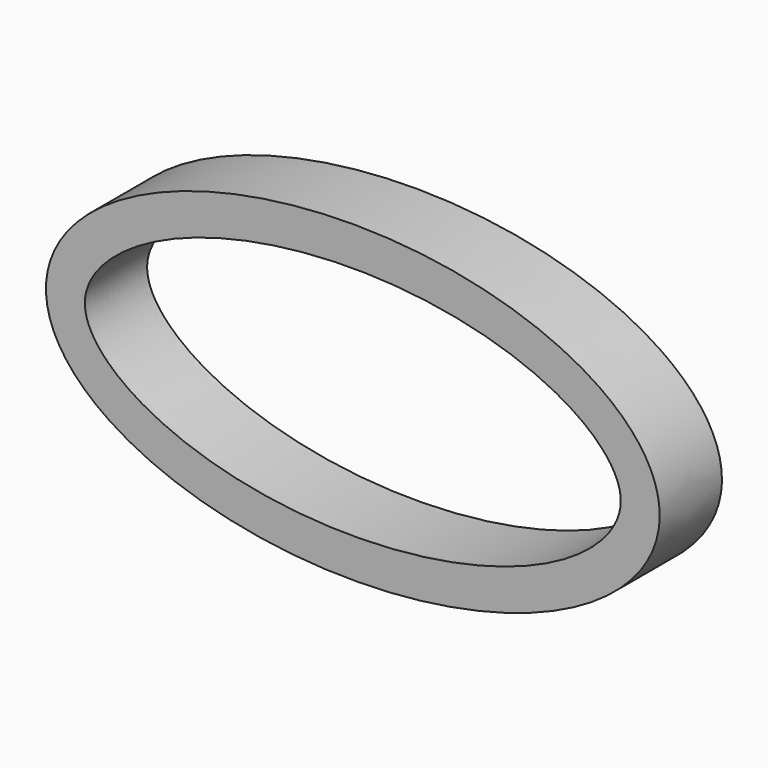
from build123d import *

# Parameters (mm, degrees)
F1_DEPTH = 12.7


# Not quite as in the source:
# - the dataset's text gives a spline's control points without its knots; the knots are read off the source's solid


with BuildPart() as f1:
    # F0 (on Front) → F1 (new body)
    with BuildSketch(Plane.XZ):
        with BuildLine():
            add(Edge.make_bspline(
                [(-50.0709774524, 20.9593381733), (-50.0709774524, -4.6166274828), (0, -4.6166274828), (50.0709774524, -4.6166274828), (50.0709774524, 20.9593381733)],
                knots=[3.1415926536, 3.1415926536, 3.1415926536, 4.7123889804, 4.7123889804, 6.2831853072, 6.2831853072, 6.2831853072], degree=2, weights=[1, 0.7071067812, 1, 0.7071067812, 1]))
            add(Edge.make_bspline(
                [(50.0709774524, 20.9593381733), (50.0709774524, 46.5353038293), (0, 46.5353038293), (-50.0709774524, 46.5353038293), (-50.0709774524, 20.9593381733)],
                knots=[0, 0, 0, 1.5707963268, 1.5707963268, 3.1415926536, 3.1415926536, 3.1415926536], degree=2, weights=[1, 0.7071067812, 1, 0.7071067812, 1]))
        make_face()
        with BuildLine():
            add(Edge.make_bspline(
                [(43.7209792435, 20.9593381733), (43.7209792435, 21.3941472691), (43.6378753479, 22.2637654609), (43.2418012763, 23.6381973689), (42.5148002756, 25.1317105062), (41.3984450909, 26.7351645875), (39.8553329616, 28.4111151874), (37.8704569502, 30.1115948), (35.8483113142, 31.5105625364), (34.0156886195, 32.5978275083), (32.5329973261, 33.3940879703), (30.9542874849, 34.1615740967), (28.741284138, 35.135430875), (25.7779291071, 36.2562859365), (21.9471588703, 37.4272897947), (17.8798753761, 38.4094991021), (13.6145661437, 39.1902890225), (9.1893604501, 39.7590330821), (5.3990551476, 40.0486007433), (2.3252694229, 40.1656128335), (0, 40.1951520139), (-2.3252694229, 40.1656128335), (-5.3990551476, 40.0486007433), (-9.1893604501, 39.7590330821), (-13.6145661437, 39.1902890225), (-17.8798753761, 38.4094991021), (-21.9471588703, 37.4272897947), (-25.7779291071, 36.2562859365), (-28.741284138, 35.135430875), (-30.9542874849, 34.1615740967), (-32.5329973261, 33.3940879703), (-34.0156886195, 32.5978275083), (-35.8483113142, 31.5105625364), (-37.8704569502, 30.1115948), (-39.8553329616, 28.4111151874), (-41.3984450909, 26.7351645875), (-42.5148002756, 25.1317105062), (-43.2418012763, 23.6381973689), (-43.6378753479, 22.2637654609), (-43.7625311913, 20.9593381733), (-43.6378753479, 19.6549108857), (-43.2418012763, 18.2804789776), (-42.5148002756, 16.7869658404), (-41.3984450909, 15.183511759), (-39.8553329616, 13.5075611592), (-37.8704569502, 11.8070815465), (-35.8483113142, 10.4081138101), (-34.0156886195, 9.3208488383), (-32.5329973261, 8.5245883762), (-30.9542874849, 7.7571022498), (-28.741284138, 6.7832454715), (-25.7779291071, 5.66239041), (-21.9471588703, 4.4913865518), (-17.8798753761, 3.5091772444), (-13.6145661437, 2.7283873241), (-9.1893604501, 2.1596432645), (-5.3990551476, 1.8700756033), (-2.3252694229, 1.753063513), (0, 1.7235243327), (2.3252694229, 1.753063513), (5.3990551476, 1.8700756033), (9.1893604501, 2.1596432645), (13.6145661437, 2.7283873241), (17.8798753761, 3.5091772444), (21.9471588703, 4.4913865518), (25.7779291071, 5.66239041), (28.741284138, 6.7832454715), (30.9542874849, 7.7571022498), (32.5329973261, 8.5245883762), (34.0156886195, 9.3208488383), (35.8483113142, 10.4081138101), (37.8704569502, 11.8070815465), (39.8553329616, 13.5075611592), (41.3984450909, 15.183511759), (42.5148002756, 16.7869658404), (43.2418012763, 18.2804789776), (43.6378753479, 19.6549108857), (43.7209792435, 20.5245290774), (43.7209792435, 20.9593381733)],
                knots=[0, 0, 0, 0, 0.015625, 0.03125, 0.046875, 0.0625, 0.078125, 0.09375, 0.109375, 0.1171875, 0.125, 0.1328125, 0.140625, 0.15625, 0.171875, 0.1875, 0.203125, 0.21875, 0.234375, 0.2421875, 0.25, 0.2578125, 0.265625, 0.28125, 0.296875, 0.3125, 0.328125, 0.34375, 0.359375, 0.3671875, 0.375, 0.3828125, 0.390625, 0.40625, 0.421875, 0.4375, 0.453125, 0.46875, 0.484375, 0.5, 0.515625, 0.53125, 0.546875, 0.5625, 0.578125, 0.59375, 0.609375, 0.6171875, 0.625, 0.6328125, 0.640625, 0.65625, 0.671875, 0.6875, 0.703125, 0.71875, 0.734375, 0.7421875, 0.75, 0.7578125, 0.765625, 0.78125, 0.796875, 0.8125, 0.828125, 0.84375, 0.859375, 0.8671875, 0.875, 0.8828125, 0.890625, 0.90625, 0.921875, 0.9375, 0.953125, 0.96875, 0.984375, 1, 1, 1, 1], degree=3))
        make_face(mode=Mode.SUBTRACT)
    extrude(amount=F1_DEPTH)


solid = f1.part
